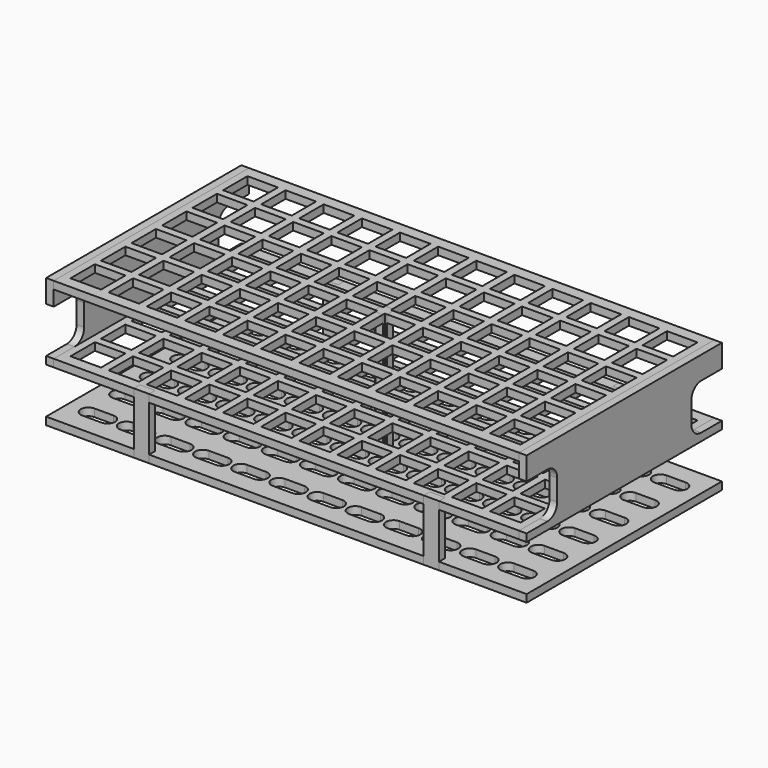
from build123d import *

# Parameters (mm, degrees)
F0_W      = 200.025
F0_H      = 101.6
F0_W_2    = 12.7
F0_H_2    = 12.7
F1_DEPTH  = 3.175
F3_W      = 200.025
F3_H      = 101.6
F3_W_2    = 12.7
F3_H_2    = 12.7
F4_DEPTH  = 3.175
F6_W      = 200.025
F6_H      = 101.6
F7_DEPTH  = 3.175
F9_DEPTH  = 3.175
F11_R     = 5.08
F11_2_R   = 5.08
F12_W     = 6.35
F12_H     = 25.4
F13_DEPTH = 3.175
F15_W     = 0.9525
F15_H     = 3.175
F15_W_2   = 3.175
F15_H_2   = 0.9525
F16_DEPTH = 50.8


# Not quite as in the source:
# - a length typed as a fraction of an inch, garbled in the dataset ("3 / 203.2 mm" for 3/8 in), is restored


with BuildPart() as f1:
    # F0 (on Top) → F1 (new body)
    with BuildSketch(Plane.XY):
        Rectangle(F0_W, F0_H)
        with Locations((-87.3125, -39.6875)):
            Rectangle(F0_W_2, F0_H_2, mode=Mode.SUBTRACT)
        with Locations((-71.4375, -39.6875)):
            Rectangle(F0_W_2, F0_H_2, mode=Mode.SUBTRACT)
        with Locations((-55.5625, -39.6875)):
            Rectangle(F0_W_2, F0_H_2, mode=Mode.SUBTRACT)
        with Locations((-39.6875, -39.6875)):
            Rectangle(F0_W_2, F0_H_2, mode=Mode.SUBTRACT)
        with Locations((-23.8125, -39.6875)):
            Rectangle(F0_W_2, F0_H_2, mode=Mode.SUBTRACT)
        with Locations((-7.9375, -39.6875)):
            Rectangle(F0_W_2, F0_H_2, mode=Mode.SUBTRACT)
        with Locations((-87.3125, -23.8125)):
            Rectangle(F0_W_2, F0_H_2, mode=Mode.SUBTRACT)
        with Locations((-71.4375, -23.8125)):
            Rectangle(F0_W_2, F0_H_2, mode=Mode.SUBTRACT)
        with Locations((-55.5625, -23.8125)):
            Rectangle(F0_W_2, F0_H_2, mode=Mode.SUBTRACT)
        with Locations((-87.3125, -7.9375)):
            Rectangle(F0_W_2, F0_H_2, mode=Mode.SUBTRACT)
        with Locations((-71.4375, -7.9375)):
            Rectangle(F0_W_2, F0_H_2, mode=Mode.SUBTRACT)
        with Locations((-55.5625, -7.9375)):
            Rectangle(F0_W_2, F0_H_2, mode=Mode.SUBTRACT)
        with Locations((-39.6875, -23.8125)):
            Rectangle(F0_W_2, F0_H_2, mode=Mode.SUBTRACT)
        with Locations((-23.8125, -23.8125)):
            Rectangle(F0_W_2, F0_H_2, mode=Mode.SUBTRACT)
        with Locations((-7.9375, -23.8125)):
            Rectangle(F0_W_2, F0_H_2, mode=Mode.SUBTRACT)
        with Locations((-39.6875, -7.9375)):
            Rectangle(F0_W_2, F0_H_2, mode=Mode.SUBTRACT)
        with Locations((-23.8125, -7.9375)):
            Rectangle(F0_W_2, F0_H_2, mode=Mode.SUBTRACT)
        with Locations((-7.9375, -7.9375)):
            Rectangle(F0_W_2, F0_H_2, mode=Mode.SUBTRACT)
        with Locations((7.9375, -39.6875)):
            Rectangle(F0_W_2, F0_H_2, mode=Mode.SUBTRACT)
        with Locations((23.8125, -39.6875)):
            Rectangle(F0_W_2, F0_H_2, mode=Mode.SUBTRACT)
        with Locations((39.6875, -39.6875)):
            Rectangle(F0_W_2, F0_H_2, mode=Mode.SUBTRACT)
        with Locations((55.5625, -39.6875)):
            Rectangle(F0_W_2, F0_H_2, mode=Mode.SUBTRACT)
        with Locations((71.4375, -39.6875)):
            Rectangle(F0_W_2, F0_H_2, mode=Mode.SUBTRACT)
        with Locations((87.3125, -39.6875)):
            Rectangle(F0_W_2, F0_H_2, mode=Mode.SUBTRACT)
        with Locations((7.9375, -23.8125)):
            Rectangle(F0_W_2, F0_H_2, mode=Mode.SUBTRACT)
        with Locations((23.8125, -23.8125)):
            Rectangle(F0_W_2, F0_H_2, mode=Mode.SUBTRACT)
        with Locations((39.6875, -23.8125)):
            Rectangle(F0_W_2, F0_H_2, mode=Mode.SUBTRACT)
        with Locations((7.9375, -7.9375)):
            Rectangle(F0_W_2, F0_H_2, mode=Mode.SUBTRACT)
        with Locations((23.8125, -7.9375)):
            Rectangle(F0_W_2, F0_H_2, mode=Mode.SUBTRACT)
        with Locations((39.6875, -7.9375)):
            Rectangle(F0_W_2, F0_H_2, mode=Mode.SUBTRACT)
        with Locations((55.5625, -23.8125)):
            Rectangle(F0_W_2, F0_H_2, mode=Mode.SUBTRACT)
        with Locations((71.4375, -23.8125)):
            Rectangle(F0_W_2, F0_H_2, mode=Mode.SUBTRACT)
        with Locations((87.3125, -23.8125)):
            Rectangle(F0_W_2, F0_H_2, mode=Mode.SUBTRACT)
        with Locations((55.5625, -7.9375)):
            Rectangle(F0_W_2, F0_H_2, mode=Mode.SUBTRACT)
        with Locations((71.4375, -7.9375)):
            Rectangle(F0_W_2, F0_H_2, mode=Mode.SUBTRACT)
        with Locations((87.3125, -7.9375)):
            Rectangle(F0_W_2, F0_H_2, mode=Mode.SUBTRACT)
        with Locations((-87.3125, 7.9375)):
            Rectangle(F0_W_2, F0_H_2, mode=Mode.SUBTRACT)
        with Locations((-71.4375, 7.9375)):
            Rectangle(F0_W_2, F0_H_2, mode=Mode.SUBTRACT)
        with Locations((-55.5625, 7.9375)):
            Rectangle(F0_W_2, F0_H_2, mode=Mode.SUBTRACT)
        with Locations((-87.3125, 23.8125)):
            Rectangle(F0_W_2, F0_H_2, mode=Mode.SUBTRACT)
        with Locations((-71.4375, 23.8125)):
            Rectangle(F0_W_2, F0_H_2, mode=Mode.SUBTRACT)
        with Locations((-55.5625, 23.8125)):
            Rectangle(F0_W_2, F0_H_2, mode=Mode.SUBTRACT)
        with Locations((-39.6875, 7.9375)):
            Rectangle(F0_W_2, F0_H_2, mode=Mode.SUBTRACT)
        with Locations((-23.8125, 7.9375)):
            Rectangle(F0_W_2, F0_H_2, mode=Mode.SUBTRACT)
        with Locations((-7.9375, 7.9375)):
            Rectangle(F0_W_2, F0_H_2, mode=Mode.SUBTRACT)
        with Locations((-39.6875, 23.8125)):
            Rectangle(F0_W_2, F0_H_2, mode=Mode.SUBTRACT)
        with Locations((-23.8125, 23.8125)):
            Rectangle(F0_W_2, F0_H_2, mode=Mode.SUBTRACT)
        with Locations((-7.9375, 23.8125)):
            Rectangle(F0_W_2, F0_H_2, mode=Mode.SUBTRACT)
        with Locations((-87.3125, 39.6875)):
            Rectangle(F0_W_2, F0_H_2, mode=Mode.SUBTRACT)
        with Locations((-71.4375, 39.6875)):
            Rectangle(F0_W_2, F0_H_2, mode=Mode.SUBTRACT)
        with Locations((-55.5625, 39.6875)):
            Rectangle(F0_W_2, F0_H_2, mode=Mode.SUBTRACT)
        with Locations((-39.6875, 39.6875)):
            Rectangle(F0_W_2, F0_H_2, mode=Mode.SUBTRACT)
        with Locations((-23.8125, 39.6875)):
            Rectangle(F0_W_2, F0_H_2, mode=Mode.SUBTRACT)
        with Locations((-7.9375, 39.6875)):
            Rectangle(F0_W_2, F0_H_2, mode=Mode.SUBTRACT)
        with Locations((7.9375, 7.9375)):
            Rectangle(F0_W_2, F0_H_2, mode=Mode.SUBTRACT)
        with Locations((23.8125, 7.9375)):
            Rectangle(F0_W_2, F0_H_2, mode=Mode.SUBTRACT)
        with Locations((39.6875, 7.9375)):
            Rectangle(F0_W_2, F0_H_2, mode=Mode.SUBTRACT)
        with Locations((7.9375, 23.8125)):
            Rectangle(F0_W_2, F0_H_2, mode=Mode.SUBTRACT)
        with Locations((23.8125, 23.8125)):
            Rectangle(F0_W_2, F0_H_2, mode=Mode.SUBTRACT)
        with Locations((39.6875, 23.8125)):
            Rectangle(F0_W_2, F0_H_2, mode=Mode.SUBTRACT)
        with Locations((55.5625, 7.9375)):
            Rectangle(F0_W_2, F0_H_2, mode=Mode.SUBTRACT)
        with Locations((71.4375, 7.9375)):
            Rectangle(F0_W_2, F0_H_2, mode=Mode.SUBTRACT)
        with Locations((87.3125, 7.9375)):
            Rectangle(F0_W_2, F0_H_2, mode=Mode.SUBTRACT)
        with Locations((55.5625, 23.8125)):
            Rectangle(F0_W_2, F0_H_2, mode=Mode.SUBTRACT)
        with Locations((71.4375, 23.8125)):
            Rectangle(F0_W_2, F0_H_2, mode=Mode.SUBTRACT)
        with Locations((87.3125, 23.8125)):
            Rectangle(F0_W_2, F0_H_2, mode=Mode.SUBTRACT)
        with Locations((7.9375, 39.6875)):
            Rectangle(F0_W_2, F0_H_2, mode=Mode.SUBTRACT)
        with Locations((23.8125, 39.6875)):
            Rectangle(F0_W_2, F0_H_2, mode=Mode.SUBTRACT)
        with Locations((39.6875, 39.6875)):
            Rectangle(F0_W_2, F0_H_2, mode=Mode.SUBTRACT)
        with Locations((55.5625, 39.6875)):
            Rectangle(F0_W_2, F0_H_2, mode=Mode.SUBTRACT)
        with Locations((71.4375, 39.6875)):
            Rectangle(F0_W_2, F0_H_2, mode=Mode.SUBTRACT)
        with Locations((87.3125, 39.6875)):
            Rectangle(F0_W_2, F0_H_2, mode=Mode.SUBTRACT)
    extrude(amount=-F1_DEPTH)


with BuildPart() as f4:
    # F3 (on offset) → F4 (new body)
    with BuildSketch(Plane.XY.offset(25.4)):
        Rectangle(F3_W, F3_H)
        with Locations((-87.3125, -39.6875)):
            Rectangle(F3_W_2, F3_H_2, mode=Mode.SUBTRACT)
        with Locations((-71.4375, -39.6875)):
            Rectangle(F3_W_2, F3_H_2, mode=Mode.SUBTRACT)
        with Locations((-55.5625, -39.6875)):
            Rectangle(F3_W_2, F3_H_2, mode=Mode.SUBTRACT)
        with Locations((-39.6875, -39.6875)):
            Rectangle(F3_W_2, F3_H_2, mode=Mode.SUBTRACT)
        with Locations((-23.8125, -39.6875)):
            Rectangle(F3_W_2, F3_H_2, mode=Mode.SUBTRACT)
        with Locations((-7.9375, -39.6875)):
            Rectangle(F3_W_2, F3_H_2, mode=Mode.SUBTRACT)
        with Locations((-87.3125, -23.8125)):
            Rectangle(F3_W_2, F3_H_2, mode=Mode.SUBTRACT)
        with Locations((-71.4375, -23.8125)):
            Rectangle(F3_W_2, F3_H_2, mode=Mode.SUBTRACT)
        with Locations((-55.5625, -23.8125)):
            Rectangle(F3_W_2, F3_H_2, mode=Mode.SUBTRACT)
        with Locations((-87.3125, -7.9375)):
            Rectangle(F3_W_2, F3_H_2, mode=Mode.SUBTRACT)
        with Locations((-71.4375, -7.9375)):
            Rectangle(F3_W_2, F3_H_2, mode=Mode.SUBTRACT)
        with Locations((-55.5625, -7.9375)):
            Rectangle(F3_W_2, F3_H_2, mode=Mode.SUBTRACT)
        with Locations((-39.6875, -23.8125)):
            Rectangle(F3_W_2, F3_H_2, mode=Mode.SUBTRACT)
        with Locations((-23.8125, -23.8125)):
            Rectangle(F3_W_2, F3_H_2, mode=Mode.SUBTRACT)
        with Locations((-7.9375, -23.8125)):
            Rectangle(F3_W_2, F3_H_2, mode=Mode.SUBTRACT)
        with Locations((-39.6875, -7.9375)):
            Rectangle(F3_W_2, F3_H_2, mode=Mode.SUBTRACT)
        with Locations((-23.8125, -7.9375)):
            Rectangle(F3_W_2, F3_H_2, mode=Mode.SUBTRACT)
        with Locations((-7.9375, -7.9375)):
            Rectangle(F3_W_2, F3_H_2, mode=Mode.SUBTRACT)
        with Locations((7.9375, -39.6875)):
            Rectangle(F3_W_2, F3_H_2, mode=Mode.SUBTRACT)
        with Locations((23.8125, -39.6875)):
            Rectangle(F3_W_2, F3_H_2, mode=Mode.SUBTRACT)
        with Locations((39.6875, -39.6875)):
            Rectangle(F3_W_2, F3_H_2, mode=Mode.SUBTRACT)
        with Locations((55.5625, -39.6875)):
            Rectangle(F3_W_2, F3_H_2, mode=Mode.SUBTRACT)
        with Locations((71.4375, -39.6875)):
            Rectangle(F3_W_2, F3_H_2, mode=Mode.SUBTRACT)
        with Locations((87.3125, -39.6875)):
            Rectangle(F3_W_2, F3_H_2, mode=Mode.SUBTRACT)
        with Locations((7.9375, -23.8125)):
            Rectangle(F3_W_2, F3_H_2, mode=Mode.SUBTRACT)
        with Locations((23.8125, -23.8125)):
            Rectangle(F3_W_2, F3_H_2, mode=Mode.SUBTRACT)
        with Locations((39.6875, -23.8125)):
            Rectangle(F3_W_2, F3_H_2, mode=Mode.SUBTRACT)
        with Locations((7.9375, -7.9375)):
            Rectangle(F3_W_2, F3_H_2, mode=Mode.SUBTRACT)
        with Locations((23.8125, -7.9375)):
            Rectangle(F3_W_2, F3_H_2, mode=Mode.SUBTRACT)
        with Locations((39.6875, -7.9375)):
            Rectangle(F3_W_2, F3_H_2, mode=Mode.SUBTRACT)
        with Locations((55.5625, -23.8125)):
            Rectangle(F3_W_2, F3_H_2, mode=Mode.SUBTRACT)
        with Locations((71.4375, -23.8125)):
            Rectangle(F3_W_2, F3_H_2, mode=Mode.SUBTRACT)
        with Locations((87.3125, -23.8125)):
            Rectangle(F3_W_2, F3_H_2, mode=Mode.SUBTRACT)
        with Locations((55.5625, -7.9375)):
            Rectangle(F3_W_2, F3_H_2, mode=Mode.SUBTRACT)
        with Locations((71.4375, -7.9375)):
            Rectangle(F3_W_2, F3_H_2, mode=Mode.SUBTRACT)
        with Locations((87.3125, -7.9375)):
            Rectangle(F3_W_2, F3_H_2, mode=Mode.SUBTRACT)
        with Locations((-87.3125, 7.9375)):
            Rectangle(F3_W_2, F3_H_2, mode=Mode.SUBTRACT)
        with Locations((-71.4375, 7.9375)):
            Rectangle(F3_W_2, F3_H_2, mode=Mode.SUBTRACT)
        with Locations((-55.5625, 7.9375)):
            Rectangle(F3_W_2, F3_H_2, mode=Mode.SUBTRACT)
        with Locations((-87.3125, 23.8125)):
            Rectangle(F3_W_2, F3_H_2, mode=Mode.SUBTRACT)
        with Locations((-71.4375, 23.8125)):
            Rectangle(F3_W_2, F3_H_2, mode=Mode.SUBTRACT)
        with Locations((-55.5625, 23.8125)):
            Rectangle(F3_W_2, F3_H_2, mode=Mode.SUBTRACT)
        with Locations((-39.6875, 7.9375)):
            Rectangle(F3_W_2, F3_H_2, mode=Mode.SUBTRACT)
        with Locations((-23.8125, 7.9375)):
            Rectangle(F3_W_2, F3_H_2, mode=Mode.SUBTRACT)
        with Locations((-7.9375, 7.9375)):
            Rectangle(F3_W_2, F3_H_2, mode=Mode.SUBTRACT)
        with Locations((-39.6875, 23.8125)):
            Rectangle(F3_W_2, F3_H_2, mode=Mode.SUBTRACT)
        with Locations((-23.8125, 23.8125)):
            Rectangle(F3_W_2, F3_H_2, mode=Mode.SUBTRACT)
        with Locations((-7.9375, 23.8125)):
            Rectangle(F3_W_2, F3_H_2, mode=Mode.SUBTRACT)
        with Locations((-87.3125, 39.6875)):
            Rectangle(F3_W_2, F3_H_2, mode=Mode.SUBTRACT)
        with Locations((-71.4375, 39.6875)):
            Rectangle(F3_W_2, F3_H_2, mode=Mode.SUBTRACT)
        with Locations((-55.5625, 39.6875)):
            Rectangle(F3_W_2, F3_H_2, mode=Mode.SUBTRACT)
        with Locations((-39.6875, 39.6875)):
            Rectangle(F3_W_2, F3_H_2, mode=Mode.SUBTRACT)
        with Locations((-23.8125, 39.6875)):
            Rectangle(F3_W_2, F3_H_2, mode=Mode.SUBTRACT)
        with Locations((-7.9375, 39.6875)):
            Rectangle(F3_W_2, F3_H_2, mode=Mode.SUBTRACT)
        with Locations((7.9375, 7.9375)):
            Rectangle(F3_W_2, F3_H_2, mode=Mode.SUBTRACT)
        with Locations((23.8125, 7.9375)):
            Rectangle(F3_W_2, F3_H_2, mode=Mode.SUBTRACT)
        with Locations((39.6875, 7.9375)):
            Rectangle(F3_W_2, F3_H_2, mode=Mode.SUBTRACT)
        with Locations((7.9375, 23.8125)):
            Rectangle(F3_W_2, F3_H_2, mode=Mode.SUBTRACT)
        with Locations((23.8125, 23.8125)):
            Rectangle(F3_W_2, F3_H_2, mode=Mode.SUBTRACT)
        with Locations((39.6875, 23.8125)):
            Rectangle(F3_W_2, F3_H_2, mode=Mode.SUBTRACT)
        with Locations((55.5625, 7.9375)):
            Rectangle(F3_W_2, F3_H_2, mode=Mode.SUBTRACT)
        with Locations((71.4375, 7.9375)):
            Rectangle(F3_W_2, F3_H_2, mode=Mode.SUBTRACT)
        with Locations((87.3125, 7.9375)):
            Rectangle(F3_W_2, F3_H_2, mode=Mode.SUBTRACT)
        with Locations((55.5625, 23.8125)):
            Rectangle(F3_W_2, F3_H_2, mode=Mode.SUBTRACT)
        with Locations((71.4375, 23.8125)):
            Rectangle(F3_W_2, F3_H_2, mode=Mode.SUBTRACT)
        with Locations((87.3125, 23.8125)):
            Rectangle(F3_W_2, F3_H_2, mode=Mode.SUBTRACT)
        with Locations((7.9375, 39.6875)):
            Rectangle(F3_W_2, F3_H_2, mode=Mode.SUBTRACT)
        with Locations((23.8125, 39.6875)):
            Rectangle(F3_W_2, F3_H_2, mode=Mode.SUBTRACT)
        with Locations((39.6875, 39.6875)):
            Rectangle(F3_W_2, F3_H_2, mode=Mode.SUBTRACT)
        with Locations((55.5625, 39.6875)):
            Rectangle(F3_W_2, F3_H_2, mode=Mode.SUBTRACT)
        with Locations((71.4375, 39.6875)):
            Rectangle(F3_W_2, F3_H_2, mode=Mode.SUBTRACT)
        with Locations((87.3125, 39.6875)):
            Rectangle(F3_W_2, F3_H_2, mode=Mode.SUBTRACT)
    extrude(amount=F4_DEPTH)


with BuildPart() as f7:
    # F6 (on offset) → F7 (new body)
    with BuildSketch(Plane.XY.offset(-25.4)):
        Rectangle(F6_W, F6_H)
        with BuildLine():
            Line((-91.28125, -36.5125), (-83.34375, -36.5125))
            ThreePointArc((-83.34375, -36.5125), (-80.16875, -39.6875), (-83.34375, -42.8625))
            Line((-83.34375, -42.8625), (-91.28125, -42.8625))
            ThreePointArc((-91.28125, -42.8625), (-94.45625, -39.6875), (-91.28125, -36.5125))
        make_face(mode=Mode.SUBTRACT)
        with BuildLine():
            Line((-75.40625, -36.5125), (-67.46875, -36.5125))
            ThreePointArc((-67.46875, -36.5125), (-64.29375, -39.6875), (-67.46875, -42.8625))
            Line((-67.46875, -42.8625), (-75.40625, -42.8625))
            ThreePointArc((-75.40625, -42.8625), (-78.58125, -39.6875), (-75.40625, -36.5125))
        make_face(mode=Mode.SUBTRACT)
        with BuildLine():
            Line((-59.53125, -36.5125), (-51.59375, -36.5125))
            ThreePointArc((-51.59375, -36.5125), (-48.41875, -39.6875), (-51.59375, -42.8625))
            Line((-51.59375, -42.8625), (-59.53125, -42.8625))
            ThreePointArc((-59.53125, -42.8625), (-62.70625, -39.6875), (-59.53125, -36.5125))
        make_face(mode=Mode.SUBTRACT)
        with BuildLine():
            Line((-43.65625, -36.5125), (-35.71875, -36.5125))
            ThreePointArc((-35.71875, -36.5125), (-32.54375, -39.6875), (-35.71875, -42.8625))
            Line((-35.71875, -42.8625), (-43.65625, -42.8625))
            ThreePointArc((-43.65625, -42.8625), (-46.83125, -39.6875), (-43.65625, -36.5125))
        make_face(mode=Mode.SUBTRACT)
        with BuildLine():
            Line((-27.78125, -36.5125), (-19.84375, -36.5125))
            ThreePointArc((-19.84375, -36.5125), (-16.66875, -39.6875), (-19.84375, -42.8625))
            Line((-19.84375, -42.8625), (-27.78125, -42.8625))
            ThreePointArc((-27.78125, -42.8625), (-30.95625, -39.6875), (-27.78125, -36.5125))
        make_face(mode=Mode.SUBTRACT)
        with BuildLine():
            Line((-11.90625, -36.5125), (-3.96875, -36.5125))
            ThreePointArc((-3.96875, -36.5125), (-0.79375, -39.6875), (-3.96875, -42.8625))
            Line((-3.96875, -42.8625), (-11.90625, -42.8625))
            ThreePointArc((-11.90625, -42.8625), (-15.08125, -39.6875), (-11.90625, -36.5125))
        make_face(mode=Mode.SUBTRACT)
        with BuildLine():
            Line((-91.28125, -20.6375), (-83.34375, -20.6375))
            ThreePointArc((-83.34375, -20.6375), (-80.16875, -23.8125), (-83.34375, -26.9875))
            Line((-83.34375, -26.9875), (-91.28125, -26.9875))
            ThreePointArc((-91.28125, -26.9875), (-94.45625, -23.8125), (-91.28125, -20.6375))
        make_face(mode=Mode.SUBTRACT)
        with BuildLine():
            Line((-75.40625, -20.6375), (-67.46875, -20.6375))
            ThreePointArc((-67.46875, -20.6375), (-64.29375, -23.8125), (-67.46875, -26.9875))
            Line((-67.46875, -26.9875), (-75.40625, -26.9875))
            ThreePointArc((-75.40625, -26.9875), (-78.58125, -23.8125), (-75.40625, -20.6375))
        make_face(mode=Mode.SUBTRACT)
        with BuildLine():
            Line((-59.53125, -20.6375), (-51.59375, -20.6375))
            ThreePointArc((-51.59375, -20.6375), (-48.41875, -23.8125), (-51.59375, -26.9875))
            Line((-51.59375, -26.9875), (-59.53125, -26.9875))
            ThreePointArc((-59.53125, -26.9875), (-62.70625, -23.8125), (-59.53125, -20.6375))
        make_face(mode=Mode.SUBTRACT)
        with BuildLine():
            Line((-91.28125, -4.7625), (-83.34375, -4.7625))
            ThreePointArc((-83.34375, -4.7625), (-80.16875, -7.9375), (-83.34375, -11.1125))
            Line((-83.34375, -11.1125), (-91.28125, -11.1125))
            ThreePointArc((-91.28125, -11.1125), (-94.45625, -7.9375), (-91.28125, -4.7625))
        make_face(mode=Mode.SUBTRACT)
        with BuildLine():
            Line((-75.40625, -4.7625), (-67.46875, -4.7625))
            ThreePointArc((-67.46875, -4.7625), (-64.29375, -7.9375), (-67.46875, -11.1125))
            Line((-67.46875, -11.1125), (-75.40625, -11.1125))
            ThreePointArc((-75.40625, -11.1125), (-78.58125, -7.9375), (-75.40625, -4.7625))
        make_face(mode=Mode.SUBTRACT)
        with BuildLine():
            Line((-59.53125, -4.7625), (-51.59375, -4.7625))
            ThreePointArc((-51.59375, -4.7625), (-48.41875, -7.9375), (-51.59375, -11.1125))
            Line((-51.59375, -11.1125), (-59.53125, -11.1125))
            ThreePointArc((-59.53125, -11.1125), (-62.70625, -7.9375), (-59.53125, -4.7625))
        make_face(mode=Mode.SUBTRACT)
        with BuildLine():
            Line((-43.65625, -20.6375), (-35.71875, -20.6375))
            ThreePointArc((-35.71875, -20.6375), (-32.54375, -23.8125), (-35.71875, -26.9875))
            Line((-35.71875, -26.9875), (-43.65625, -26.9875))
            ThreePointArc((-43.65625, -26.9875), (-46.83125, -23.8125), (-43.65625, -20.6375))
        make_face(mode=Mode.SUBTRACT)
        with BuildLine():
            Line((-27.78125, -20.6375), (-19.84375, -20.6375))
            ThreePointArc((-19.84375, -20.6375), (-16.66875, -23.8125), (-19.84375, -26.9875))
            Line((-19.84375, -26.9875), (-27.78125, -26.9875))
            ThreePointArc((-27.78125, -26.9875), (-30.95625, -23.8125), (-27.78125, -20.6375))
        make_face(mode=Mode.SUBTRACT)
        with BuildLine():
            Line((-11.90625, -20.6375), (-3.96875, -20.6375))
            ThreePointArc((-3.96875, -20.6375), (-0.79375, -23.8125), (-3.96875, -26.9875))
            Line((-3.96875, -26.9875), (-11.90625, -26.9875))
            ThreePointArc((-11.90625, -26.9875), (-15.08125, -23.8125), (-11.90625, -20.6375))
        make_face(mode=Mode.SUBTRACT)
        with BuildLine():
            Line((-43.65625, -4.7625), (-35.71875, -4.7625))
            ThreePointArc((-35.71875, -4.7625), (-32.54375, -7.9375), (-35.71875, -11.1125))
            Line((-35.71875, -11.1125), (-43.65625, -11.1125))
            ThreePointArc((-43.65625, -11.1125), (-46.83125, -7.9375), (-43.65625, -4.7625))
        make_face(mode=Mode.SUBTRACT)
        with BuildLine():
            Line((-27.78125, -4.7625), (-19.84375, -4.7625))
            ThreePointArc((-19.84375, -4.7625), (-16.66875, -7.9375), (-19.84375, -11.1125))
            Line((-19.84375, -11.1125), (-27.78125, -11.1125))
            ThreePointArc((-27.78125, -11.1125), (-30.95625, -7.9375), (-27.78125, -4.7625))
        make_face(mode=Mode.SUBTRACT)
        with BuildLine():
            Line((-11.90625, -4.7625), (-7.9375, -4.7625))
            Line((-7.9375, -4.7625), (-3.96875, -4.7625))
            ThreePointArc((-3.96875, -4.7625), (-0.79375, -7.9375), (-3.96875, -11.1125))
            Line((-3.96875, -11.1125), (-11.90625, -11.1125))
            ThreePointArc((-11.90625, -11.1125), (-15.08125, -7.9375), (-11.90625, -4.7625))
        make_face(mode=Mode.SUBTRACT)
        with BuildLine():
            ThreePointArc((3.96875, -42.8625), (0.79375, -39.6875), (3.96875, -36.5125))
            Line((3.96875, -36.5125), (11.90625, -36.5125))
            ThreePointArc((11.90625, -36.5125), (15.08125, -39.6875), (11.90625, -42.8625))
            Line((11.90625, -42.8625), (3.96875, -42.8625))
        make_face(mode=Mode.SUBTRACT)
        with BuildLine():
            Line((19.84375, -36.5125), (27.78125, -36.5125))
            ThreePointArc((27.78125, -36.5125), (30.95625, -39.6875), (27.78125, -42.8625))
            Line((27.78125, -42.8625), (19.84375, -42.8625))
            ThreePointArc((19.84375, -42.8625), (16.66875, -39.6875), (19.84375, -36.5125))
        make_face(mode=Mode.SUBTRACT)
        with BuildLine():
            ThreePointArc((35.71875, -42.8625), (32.54375, -39.6875), (35.71875, -36.5125))
            Line((35.71875, -36.5125), (43.65625, -36.5125))
            ThreePointArc((43.65625, -36.5125), (46.83125, -39.6875), (43.65625, -42.8625))
            Line((43.65625, -42.8625), (35.71875, -42.8625))
        make_face(mode=Mode.SUBTRACT)
        with BuildLine():
            ThreePointArc((51.59375, -42.8625), (48.41875, -39.6875), (51.59375, -36.5125))
            Line((51.59375, -36.5125), (59.53125, -36.5125))
            ThreePointArc((59.53125, -36.5125), (62.70625, -39.6875), (59.53125, -42.8625))
            Line((59.53125, -42.8625), (51.59375, -42.8625))
        make_face(mode=Mode.SUBTRACT)
        with BuildLine():
            Line((67.46875, -36.5125), (75.40625, -36.5125))
            ThreePointArc((75.40625, -36.5125), (78.58125, -39.6875), (75.40625, -42.8625))
            Line((75.40625, -42.8625), (67.46875, -42.8625))
            ThreePointArc((67.46875, -42.8625), (64.29375, -39.6875), (67.46875, -36.5125))
        make_face(mode=Mode.SUBTRACT)
        with BuildLine():
            Line((83.34375, -36.5125), (91.28125, -36.5125))
            ThreePointArc((91.28125, -36.5125), (94.45625, -39.6875), (91.28125, -42.8625))
            Line((91.28125, -42.8625), (83.34375, -42.8625))
            ThreePointArc((83.34375, -42.8625), (80.16875, -39.6875), (83.34375, -36.5125))
        make_face(mode=Mode.SUBTRACT)
        with BuildLine():
            ThreePointArc((3.96875, -26.9875), (0.79375, -23.8125), (3.96875, -20.6375))
            Line((3.96875, -20.6375), (11.90625, -20.6375))
            ThreePointArc((11.90625, -20.6375), (15.08125, -23.8125), (11.90625, -26.9875))
            Line((11.90625, -26.9875), (3.96875, -26.9875))
        make_face(mode=Mode.SUBTRACT)
        with BuildLine():
            ThreePointArc((19.84375, -26.9875), (16.66875, -23.8125), (19.84375, -20.6375))
            Line((19.84375, -20.6375), (27.78125, -20.6375))
            ThreePointArc((27.78125, -20.6375), (30.95625, -23.8125), (27.78125, -26.9875))
            Line((27.78125, -26.9875), (19.84375, -26.9875))
        make_face(mode=Mode.SUBTRACT)
        with BuildLine():
            ThreePointArc((35.71875, -26.9875), (32.54375, -23.8125), (35.71875, -20.6375))
            Line((35.71875, -20.6375), (43.65625, -20.6375))
            ThreePointArc((43.65625, -20.6375), (46.83125, -23.8125), (43.65625, -26.9875))
            Line((43.65625, -26.9875), (35.71875, -26.9875))
        make_face(mode=Mode.SUBTRACT)
        with BuildLine():
            Line((3.96875, -4.7625), (7.9375, -4.7625))
            Line((7.9375, -4.7625), (11.90625, -4.7625))
            ThreePointArc((11.90625, -4.7625), (15.08125, -7.9375), (11.90625, -11.1125))
            Line((11.90625, -11.1125), (3.96875, -11.1125))
            ThreePointArc((3.96875, -11.1125), (0.79375, -7.9375), (3.96875, -4.7625))
        make_face(mode=Mode.SUBTRACT)
        with BuildLine():
            ThreePointArc((19.84375, -11.1125), (16.66875, -7.9375), (19.84375, -4.7625))
            Line((19.84375, -4.7625), (27.78125, -4.7625))
            ThreePointArc((27.78125, -4.7625), (30.95625, -7.9375), (27.78125, -11.1125))
            Line((27.78125, -11.1125), (19.84375, -11.1125))
        make_face(mode=Mode.SUBTRACT)
        with BuildLine():
            ThreePointArc((35.71875, -11.1125), (32.54375, -7.9375), (35.71875, -4.7625))
            Line((35.71875, -4.7625), (43.65625, -4.7625))
            ThreePointArc((43.65625, -4.7625), (46.83125, -7.9375), (43.65625, -11.1125))
            Line((43.65625, -11.1125), (35.71875, -11.1125))
        make_face(mode=Mode.SUBTRACT)
        with BuildLine():
            Line((51.59375, -20.6375), (59.53125, -20.6375))
            ThreePointArc((59.53125, -20.6375), (62.70625, -23.8125), (59.53125, -26.9875))
            Line((59.53125, -26.9875), (51.59375, -26.9875))
            ThreePointArc((51.59375, -26.9875), (48.41875, -23.8125), (51.59375, -20.6375))
        make_face(mode=Mode.SUBTRACT)
        with BuildLine():
            Line((67.46875, -20.6375), (75.40625, -20.6375))
            ThreePointArc((75.40625, -20.6375), (78.58125, -23.8125), (75.40625, -26.9875))
            Line((75.40625, -26.9875), (67.46875, -26.9875))
            ThreePointArc((67.46875, -26.9875), (64.29375, -23.8125), (67.46875, -20.6375))
        make_face(mode=Mode.SUBTRACT)
        with BuildLine():
            Line((91.28125, -26.9875), (83.34375, -26.9875))
            ThreePointArc((83.34375, -26.9875), (80.16875, -23.8125), (83.34375, -20.6375))
            Line((83.34375, -20.6375), (91.28125, -20.6375))
            ThreePointArc((91.28125, -20.6375), (94.45625, -23.8125), (91.28125, -26.9875))
        make_face(mode=Mode.SUBTRACT)
        with BuildLine():
            Line((51.59375, -4.7625), (59.53125, -4.7625))
            ThreePointArc((59.53125, -4.7625), (62.70625, -7.9375), (59.53125, -11.1125))
            Line((59.53125, -11.1125), (51.59375, -11.1125))
            ThreePointArc((51.59375, -11.1125), (48.41875, -7.9375), (51.59375, -4.7625))
        make_face(mode=Mode.SUBTRACT)
        with BuildLine():
            ThreePointArc((67.46875, -11.1125), (64.29375, -7.9375), (67.46875, -4.7625))
            Line((67.46875, -4.7625), (75.40625, -4.7625))
            ThreePointArc((75.40625, -4.7625), (78.58125, -7.9375), (75.40625, -11.1125))
            Line((75.40625, -11.1125), (67.46875, -11.1125))
        make_face(mode=Mode.SUBTRACT)
        with BuildLine():
            ThreePointArc((83.34375, -11.1125), (80.16875, -7.9375), (83.34375, -4.7625))
            Line((83.34375, -4.7625), (91.28125, -4.7625))
            ThreePointArc((91.28125, -4.7625), (94.45625, -7.9375), (91.28125, -11.1125))
            Line((91.28125, -11.1125), (83.34375, -11.1125))
        make_face(mode=Mode.SUBTRACT)
        with BuildLine():
            ThreePointArc((-83.34375, 11.1125), (-80.16875, 7.9375), (-83.34375, 4.7625))
            Line((-83.34375, 4.7625), (-91.28125, 4.7625))
            ThreePointArc((-91.28125, 4.7625), (-94.45625, 7.9375), (-91.28125, 11.1125))
            Line((-91.28125, 11.1125), (-83.34375, 11.1125))
        make_face(mode=Mode.SUBTRACT)
        with BuildLine():
            Line((-75.40625, 11.1125), (-67.46875, 11.1125))
            ThreePointArc((-67.46875, 11.1125), (-64.29375, 7.9375), (-67.46875, 4.7625))
            Line((-67.46875, 4.7625), (-75.40625, 4.7625))
            ThreePointArc((-75.40625, 4.7625), (-78.58125, 7.9375), (-75.40625, 11.1125))
        make_face(mode=Mode.SUBTRACT)
        with BuildLine():
            ThreePointArc((-51.59375, 11.1125), (-48.41875, 7.9375), (-51.59375, 4.7625))
            Line((-51.59375, 4.7625), (-59.53125, 4.7625))
            ThreePointArc((-59.53125, 4.7625), (-62.70625, 7.9375), (-59.53125, 11.1125))
            Line((-59.53125, 11.1125), (-51.59375, 11.1125))
        make_face(mode=Mode.SUBTRACT)
        with BuildLine():
            ThreePointArc((-83.34375, 26.9875), (-80.16875, 23.8125), (-83.34375, 20.6375))
            Line((-83.34375, 20.6375), (-91.28125, 20.6375))
            ThreePointArc((-91.28125, 20.6375), (-94.45625, 23.8125), (-91.28125, 26.9875))
            Line((-91.28125, 26.9875), (-83.34375, 26.9875))
        make_face(mode=Mode.SUBTRACT)
        with BuildLine():
            Line((-75.40625, 26.9875), (-67.46875, 26.9875))
            ThreePointArc((-67.46875, 26.9875), (-64.29375, 23.8125), (-67.46875, 20.6375))
            Line((-67.46875, 20.6375), (-75.40625, 20.6375))
            ThreePointArc((-75.40625, 20.6375), (-78.58125, 23.8125), (-75.40625, 26.9875))
        make_face(mode=Mode.SUBTRACT)
        with BuildLine():
            Line((-59.53125, 26.9875), (-51.59375, 26.9875))
            ThreePointArc((-51.59375, 26.9875), (-48.41875, 23.8125), (-51.59375, 20.6375))
            Line((-51.59375, 20.6375), (-59.53125, 20.6375))
            ThreePointArc((-59.53125, 20.6375), (-62.70625, 23.8125), (-59.53125, 26.9875))
        make_face(mode=Mode.SUBTRACT)
        with BuildLine():
            ThreePointArc((-35.71875, 11.1125), (-32.54375, 7.9375), (-35.71875, 4.7625))
            Line((-35.71875, 4.7625), (-43.65625, 4.7625))
            ThreePointArc((-43.65625, 4.7625), (-46.83125, 7.9375), (-43.65625, 11.1125))
            Line((-43.65625, 11.1125), (-35.71875, 11.1125))
        make_face(mode=Mode.SUBTRACT)
        with BuildLine():
            ThreePointArc((-19.84375, 11.1125), (-16.66875, 7.9375), (-19.84375, 4.7625))
            Line((-19.84375, 4.7625), (-27.78125, 4.7625))
            ThreePointArc((-27.78125, 4.7625), (-30.95625, 7.9375), (-27.78125, 11.1125))
            Line((-27.78125, 11.1125), (-19.84375, 11.1125))
        make_face(mode=Mode.SUBTRACT)
        with BuildLine():
            Line((-3.96875, 4.7625), (-11.90625, 4.7625))
            ThreePointArc((-11.90625, 4.7625), (-15.08125, 7.9375), (-11.90625, 11.1125))
            Line((-11.90625, 11.1125), (-3.96875, 11.1125))
            ThreePointArc((-3.96875, 11.1125), (-0.79375, 7.9375), (-3.96875, 4.7625))
        make_face(mode=Mode.SUBTRACT)
        with BuildLine():
            Line((-35.71875, 20.6375), (-43.65625, 20.6375))
            ThreePointArc((-43.65625, 20.6375), (-46.83125, 23.8125), (-43.65625, 26.9875))
            Line((-43.65625, 26.9875), (-35.71875, 26.9875))
            ThreePointArc((-35.71875, 26.9875), (-32.54375, 23.8125), (-35.71875, 20.6375))
        make_face(mode=Mode.SUBTRACT)
        with BuildLine():
            ThreePointArc((-19.84375, 26.9875), (-16.66875, 23.8125), (-19.84375, 20.6375))
            Line((-19.84375, 20.6375), (-27.78125, 20.6375))
            ThreePointArc((-27.78125, 20.6375), (-30.95625, 23.8125), (-27.78125, 26.9875))
            Line((-27.78125, 26.9875), (-19.84375, 26.9875))
        make_face(mode=Mode.SUBTRACT)
        with BuildLine():
            Line((-11.90625, 26.9875), (-3.96875, 26.9875))
            ThreePointArc((-3.96875, 26.9875), (-0.79375, 23.8125), (-3.96875, 20.6375))
            Line((-3.96875, 20.6375), (-11.90625, 20.6375))
            ThreePointArc((-11.90625, 20.6375), (-15.08125, 23.8125), (-11.90625, 26.9875))
        make_face(mode=Mode.SUBTRACT)
        with BuildLine():
            ThreePointArc((-83.34375, 42.8625), (-80.16875, 39.6875), (-83.34375, 36.5125))
            Line((-83.34375, 36.5125), (-91.28125, 36.5125))
            ThreePointArc((-91.28125, 36.5125), (-94.45625, 39.6875), (-91.28125, 42.8625))
            Line((-91.28125, 42.8625), (-83.34375, 42.8625))
        make_face(mode=Mode.SUBTRACT)
        with BuildLine():
            Line((-67.46875, 36.5125), (-75.40625, 36.5125))
            ThreePointArc((-75.40625, 36.5125), (-78.58125, 39.6875), (-75.40625, 42.8625))
            Line((-75.40625, 42.8625), (-67.46875, 42.8625))
            ThreePointArc((-67.46875, 42.8625), (-64.29375, 39.6875), (-67.46875, 36.5125))
        make_face(mode=Mode.SUBTRACT)
        with BuildLine():
            ThreePointArc((-51.59375, 42.8625), (-48.41875, 39.6875), (-51.59375, 36.5125))
            Line((-51.59375, 36.5125), (-59.53125, 36.5125))
            ThreePointArc((-59.53125, 36.5125), (-62.70625, 39.6875), (-59.53125, 42.8625))
            Line((-59.53125, 42.8625), (-51.59375, 42.8625))
        make_face(mode=Mode.SUBTRACT)
        with BuildLine():
            ThreePointArc((-35.71875, 42.8625), (-32.54375, 39.6875), (-35.71875, 36.5125))
            Line((-35.71875, 36.5125), (-43.65625, 36.5125))
            ThreePointArc((-43.65625, 36.5125), (-46.83125, 39.6875), (-43.65625, 42.8625))
            Line((-43.65625, 42.8625), (-35.71875, 42.8625))
        make_face(mode=Mode.SUBTRACT)
        with BuildLine():
            ThreePointArc((-19.84375, 42.8625), (-16.66875, 39.6875), (-19.84375, 36.5125))
            Line((-19.84375, 36.5125), (-27.78125, 36.5125))
            ThreePointArc((-27.78125, 36.5125), (-30.95625, 39.6875), (-27.78125, 42.8625))
            Line((-27.78125, 42.8625), (-19.84375, 42.8625))
        make_face(mode=Mode.SUBTRACT)
        with BuildLine():
            Line((-3.96875, 36.5125), (-11.90625, 36.5125))
            ThreePointArc((-11.90625, 36.5125), (-15.08125, 39.6875), (-11.90625, 42.8625))
            Line((-11.90625, 42.8625), (-3.96875, 42.8625))
            ThreePointArc((-3.96875, 42.8625), (-0.79375, 39.6875), (-3.96875, 36.5125))
        make_face(mode=Mode.SUBTRACT)
        with BuildLine():
            Line((11.90625, 4.7625), (3.96875, 4.7625))
            ThreePointArc((3.96875, 4.7625), (0.79375, 7.9375), (3.96875, 11.1125))
            Line((3.96875, 11.1125), (11.90625, 11.1125))
            ThreePointArc((11.90625, 11.1125), (15.08125, 7.9375), (11.90625, 4.7625))
        make_face(mode=Mode.SUBTRACT)
        with BuildLine():
            Line((27.78125, 4.7625), (19.84375, 4.7625))
            ThreePointArc((19.84375, 4.7625), (16.66875, 7.9375), (19.84375, 11.1125))
            Line((19.84375, 11.1125), (27.78125, 11.1125))
            ThreePointArc((27.78125, 11.1125), (30.95625, 7.9375), (27.78125, 4.7625))
        make_face(mode=Mode.SUBTRACT)
        with BuildLine():
            ThreePointArc((35.71875, 4.7625), (32.54375, 7.9375), (35.71875, 11.1125))
            Line((35.71875, 11.1125), (43.65625, 11.1125))
            ThreePointArc((43.65625, 11.1125), (46.83125, 7.9375), (43.65625, 4.7625))
            Line((43.65625, 4.7625), (35.71875, 4.7625))
        make_face(mode=Mode.SUBTRACT)
        with BuildLine():
            ThreePointArc((11.90625, 26.9875), (15.08125, 23.8125), (11.90625, 20.6375))
            Line((11.90625, 20.6375), (3.96875, 20.6375))
            ThreePointArc((3.96875, 20.6375), (0.79375, 23.8125), (3.96875, 26.9875))
            Line((3.96875, 26.9875), (11.90625, 26.9875))
        make_face(mode=Mode.SUBTRACT)
        with BuildLine():
            Line((27.78125, 20.6375), (19.84375, 20.6375))
            ThreePointArc((19.84375, 20.6375), (16.66875, 23.8125), (19.84375, 26.9875))
            Line((19.84375, 26.9875), (27.78125, 26.9875))
            ThreePointArc((27.78125, 26.9875), (30.95625, 23.8125), (27.78125, 20.6375))
        make_face(mode=Mode.SUBTRACT)
        with BuildLine():
            ThreePointArc((35.71875, 20.6375), (32.54375, 23.8125), (35.71875, 26.9875))
            Line((35.71875, 26.9875), (43.65625, 26.9875))
            ThreePointArc((43.65625, 26.9875), (46.83125, 23.8125), (43.65625, 20.6375))
            Line((43.65625, 20.6375), (35.71875, 20.6375))
        make_face(mode=Mode.SUBTRACT)
        with BuildLine():
            ThreePointArc((59.53125, 11.1125), (62.70625, 7.9375), (59.53125, 4.7625))
            Line((59.53125, 4.7625), (51.59375, 4.7625))
            ThreePointArc((51.59375, 4.7625), (48.41875, 7.9375), (51.59375, 11.1125))
            Line((51.59375, 11.1125), (59.53125, 11.1125))
        make_face(mode=Mode.SUBTRACT)
        with BuildLine():
            ThreePointArc((75.40625, 11.1125), (78.58125, 7.9375), (75.40625, 4.7625))
            Line((75.40625, 4.7625), (67.46875, 4.7625))
            ThreePointArc((67.46875, 4.7625), (64.29375, 7.9375), (67.46875, 11.1125))
            Line((67.46875, 11.1125), (75.40625, 11.1125))
        make_face(mode=Mode.SUBTRACT)
        with BuildLine():
            ThreePointArc((83.34375, 4.7625), (80.16875, 7.9375), (83.34375, 11.1125))
            Line((83.34375, 11.1125), (91.28125, 11.1125))
            ThreePointArc((91.28125, 11.1125), (94.45625, 7.9375), (91.28125, 4.7625))
            Line((91.28125, 4.7625), (83.34375, 4.7625))
        make_face(mode=Mode.SUBTRACT)
        with BuildLine():
            ThreePointArc((51.59375, 20.6375), (48.41875, 23.8125), (51.59375, 26.9875))
            Line((51.59375, 26.9875), (59.53125, 26.9875))
            ThreePointArc((59.53125, 26.9875), (62.70625, 23.8125), (59.53125, 20.6375))
            Line((59.53125, 20.6375), (51.59375, 20.6375))
        make_face(mode=Mode.SUBTRACT)
        with BuildLine():
            ThreePointArc((75.40625, 26.9875), (78.58125, 23.8125), (75.40625, 20.6375))
            Line((75.40625, 20.6375), (67.46875, 20.6375))
            ThreePointArc((67.46875, 20.6375), (64.29375, 23.8125), (67.46875, 26.9875))
            Line((67.46875, 26.9875), (75.40625, 26.9875))
        make_face(mode=Mode.SUBTRACT)
        with BuildLine():
            ThreePointArc((91.28125, 26.9875), (94.45625, 23.8125), (91.28125, 20.6375))
            Line((91.28125, 20.6375), (83.34375, 20.6375))
            ThreePointArc((83.34375, 20.6375), (80.16875, 23.8125), (83.34375, 26.9875))
            Line((83.34375, 26.9875), (91.28125, 26.9875))
        make_face(mode=Mode.SUBTRACT)
        with BuildLine():
            ThreePointArc((11.90625, 42.8625), (15.08125, 39.6875), (11.90625, 36.5125))
            Line((11.90625, 36.5125), (3.96875, 36.5125))
            ThreePointArc((3.96875, 36.5125), (0.79375, 39.6875), (3.96875, 42.8625))
            Line((3.96875, 42.8625), (11.90625, 42.8625))
        make_face(mode=Mode.SUBTRACT)
        with BuildLine():
            ThreePointArc((27.78125, 42.8625), (30.95625, 39.6875), (27.78125, 36.5125))
            Line((27.78125, 36.5125), (19.84375, 36.5125))
            ThreePointArc((19.84375, 36.5125), (16.66875, 39.6875), (19.84375, 42.8625))
            Line((19.84375, 42.8625), (27.78125, 42.8625))
        make_face(mode=Mode.SUBTRACT)
        with BuildLine():
            ThreePointArc((43.65625, 42.8625), (46.83125, 39.6875), (43.65625, 36.5125))
            Line((43.65625, 36.5125), (35.71875, 36.5125))
            ThreePointArc((35.71875, 36.5125), (32.54375, 39.6875), (35.71875, 42.8625))
            Line((35.71875, 42.8625), (43.65625, 42.8625))
        make_face(mode=Mode.SUBTRACT)
        with BuildLine():
            ThreePointArc((59.53125, 42.8625), (62.70625, 39.6875), (59.53125, 36.5125))
            Line((59.53125, 36.5125), (51.59375, 36.5125))
            ThreePointArc((51.59375, 36.5125), (48.41875, 39.6875), (51.59375, 42.8625))
            Line((51.59375, 42.8625), (59.53125, 42.8625))
        make_face(mode=Mode.SUBTRACT)
        with BuildLine():
            ThreePointArc((67.46875, 36.5125), (64.29375, 39.6875), (67.46875, 42.8625))
            Line((67.46875, 42.8625), (75.40625, 42.8625))
            ThreePointArc((75.40625, 42.8625), (78.58125, 39.6875), (75.40625, 36.5125))
            Line((75.40625, 36.5125), (67.46875, 36.5125))
        make_face(mode=Mode.SUBTRACT)
        with BuildLine():
            ThreePointArc((83.34375, 36.5125), (80.16875, 39.6875), (83.34375, 42.8625))
            Line((83.34375, 42.8625), (91.28125, 42.8625))
            ThreePointArc((91.28125, 42.8625), (94.45625, 39.6875), (91.28125, 36.5125))
            Line((91.28125, 36.5125), (83.34375, 36.5125))
        make_face(mode=Mode.SUBTRACT)
    extrude(amount=F7_DEPTH)


with BuildPart() as f9:
    # F8 (on face) → F9 (new body)
    with BuildSketch(Plane.YZ.offset(100.0125)):
        Polygon((-34.925, 0), (0, 0), (34.925, 0), (34.925, 19.05), (-34.925, 19.05), align=None)
        Polygon((34.925, 0), (0, 0), (-34.925, 0), (-50.8, 0), (-50.8, -3.175), (50.8, -3.175), (50.8, 0), align=None)
        Polygon((-34.925, 19.05), (34.925, 19.05), (50.8, 19.05), (50.8, 28.575), (-50.8, 28.575), (-50.8, 19.05), align=None)
    extrude(amount=-F9_DEPTH)


with BuildPart() as f10_1:
    # F10: instance of F9
    add(f9.part.mirror(Plane.YZ))

    # F11#2
    f11_2_edges = [f10_1.edges().sort_by_distance(p)[0] for p in [
        (-98.425, 34.925, 19.05),
        (-98.425, -34.925, 19.05),
        (-98.425, -34.925, 0),
        (-98.425, 34.925, 0),
    ]]
    fillet(f11_2_edges, radius=F11_2_R)


with BuildPart() as f9_1:
    add(f9.part)

    # F11
    f11_edges = [f9_1.edges().sort_by_distance(p)[0] for p in [
        (98.425, -34.925, 0),
        (98.425, 34.925, 0),
        (98.425, -34.925, 19.05),
        (98.425, 34.925, 19.05),
    ]]
    fillet(f11_edges, radius=F11_R)


with BuildPart() as f13:
    # F12 (on face) → F13 (new body)
    with BuildSketch(Plane.XZ.offset(50.8)):
        with Locations((-60.325, -12.7)):
            Rectangle(F12_W, F12_H)
    extrude(amount=-F13_DEPTH)


with BuildPart() as f13b:
    # F12 (on face) → F13, piece 2 (new body)
    with BuildSketch(Plane.XZ.offset(50.8)):
        with Locations((60.325, -12.7)):
            Rectangle(F12_W, F12_H)
    extrude(amount=-F13_DEPTH)


with BuildPart() as f14_1:
    # F14: instance of F13
    add(f13.part.mirror(Plane.XZ))


with BuildPart() as f14_2:
    # F14: instance of F13b
    add(f13b.part.mirror(Plane.XZ))


with BuildPart() as f16:
    # F15 (on face) → F16 (new body)
    with BuildSketch(Plane.XY.offset(28.575)):
        with Locations((2.06375, 0)):
            Rectangle(F15_W, F15_H)
        with Locations((0, -2.06375)):
            Rectangle(F15_W_2, F15_H_2)
        Rectangle(F15_W_2, F15_H)
        with Locations((-2.06375, 0)):
            Rectangle(F15_W, F15_H)
        with Locations((0, 2.06375)):
            Rectangle(F15_W_2, F15_H_2)
    extrude(amount=-F16_DEPTH)


solid = Compound([f1.part, f4.part, f7.part, f10_1.part, f9_1.part, f13.part, f13b.part, f14_1.part, f14_2.part, f16.part])
